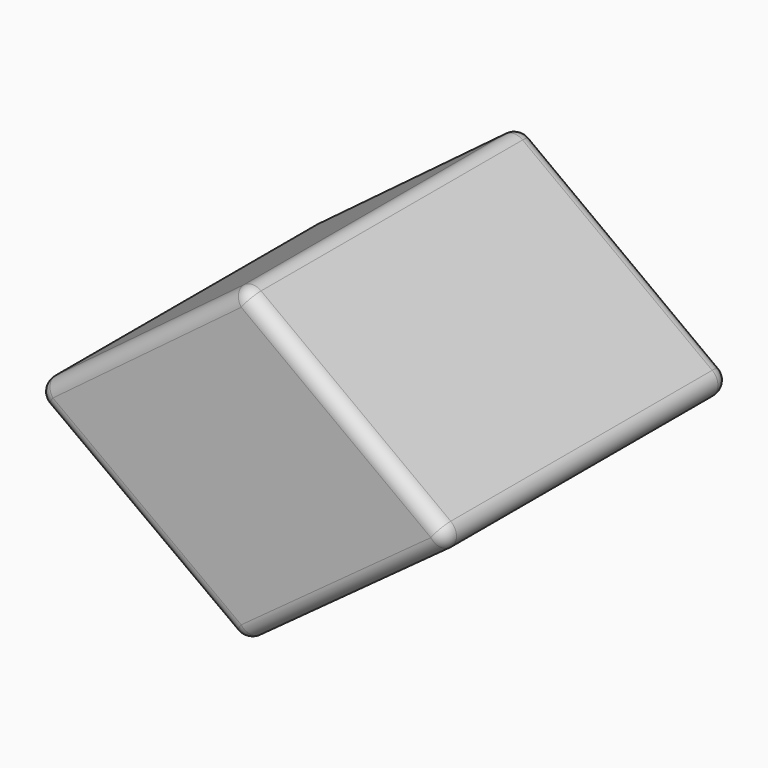
from build123d import *

# Parameters (mm, degrees)
F1_DEPTH       = 25.4
F2_R           = 15.300879685
F3_DEPTH       = 14.478
F4_DEPTH       = 101.6
F6_D           = 13.97
F6_DEPTH       = 76.2
F6_CBORE_D     = 13.97
F6_CBORE_DEPTH = 6.35
F6_TIP         = 4.1970114239
F8_D           = 13.97
F8_DEPTH       = 76.2
F8_CBORE_D     = 13.97
F8_CBORE_DEPTH = 6.35
F8_TIP         = 4.1970114239
F9_R           = 5.08


with BuildPart() as f1:
    # F0 (on Front) → F1 (new body)
    with BuildSketch(Plane.XZ):
        with BuildLine():
            ThreePointArc((-7.1662437988, 0), (-5.0672995858, 5.0672995858), (0, 7.1662437988))
            Line((0, 7.1662437988), (0, 56.8071007729))
            Line((0, 56.8071007729), (-75.8317038417, 0))
            Line((-75.8317038417, 0), (-7.1662437988, 0))
        make_face()
        with BuildLine():
            Line((0, 56.8071007729), (0, 7.1662437988))
            ThreePointArc((0, 7.1662437988), (5.0672995858, 5.0672995858), (7.1662437988, 0))
            Line((7.1662437988, 0), (76.3651058078, 0))
            Line((76.3651058078, 0), (0, 56.8071007729))
        make_face()
        with BuildLine():
            Line((76.3651058078, 0), (7.1662437988, 0))
            ThreePointArc((7.1662437988, 0), (5.0672995858, -5.0672995858), (0, -7.1662437988))
            Line((0, -7.1662437988), (0, -55.740300566))
            Line((0, -55.740300566), (76.3651058078, 0))
        make_face()
        with BuildLine():
            Line((0, -55.740300566), (0, -7.1662437988))
            ThreePointArc((0, -7.1662437988), (-5.0672995858, -5.0672995858), (-7.1662437988, 0))
            Line((-7.1662437988, 0), (-75.8317038417, 0))
            Line((-75.8317038417, 0), (0, -55.740300566))
        make_face()
        with BuildLine():
            Line((7.1662437988, 0), (0, 0))
            Line((0, 0), (0, -7.1662437988))
            ThreePointArc((0, -7.1662437988), (5.0672995858, -5.0672995858), (7.1662437988, 0))
        make_face()
        with BuildLine():
            Line((-7.1662437988, 0), (0, 0))
            Line((0, 0), (0, 7.1662437988))
            ThreePointArc((0, 7.1662437988), (-5.0672995858, 5.0672995858), (-7.1662437988, 0))
        make_face()
        with BuildLine():
            Line((0, 7.1662437988), (0, 0))
            Line((0, 0), (7.1662437988, 0))
            ThreePointArc((7.1662437988, 0), (5.0672995858, 5.0672995858), (0, 7.1662437988))
        make_face()
        with BuildLine():
            Line((0, -7.1662437988), (0, 0))
            Line((0, 0), (-7.1662437988, 0))
            ThreePointArc((-7.1662437988, 0), (-5.0672995858, -5.0672995858), (0, -7.1662437988))
        make_face()
    extrude(amount=F1_DEPTH)

    # F2 (on Front) → F3 (cut)
    with BuildSketch(Plane.XZ):
        Circle(F2_R)
    extrude(amount=F3_DEPTH, mode=Mode.SUBTRACT)

    # F4 (add): a face of the model
    f4_faces = [f1.faces().sort_by_distance(p)[0] for p in [
        (-36.7809633217, 0, 26.8885894929),
    ]]
    extrude(f4_faces, amount=F4_DEPTH)

    # F6
    with Locations(Plane(origin=(0, 101.6, 0), x_dir=(-1, 0, 0), z_dir=(0, 1, 0))):
        with Locations((-45.5900207162, 0)):
            CounterBoreHole(F6_D / 2, F6_CBORE_D / 2, F6_CBORE_DEPTH, depth=F6_DEPTH)
            with Locations((0, 0, -(F6_DEPTH + F6_TIP / 2))):  # 118° drill point
                Cone(0, F6_D / 2, F6_TIP, mode=Mode.SUBTRACT)

    # F8
    with Locations(Plane(origin=(0, 101.6, 0), x_dir=(-1, 0, 0), z_dir=(0, 1, 0))):
        with Locations((45.3492924571, 0)):
            CounterBoreHole(F8_D / 2, F8_CBORE_D / 2, F8_CBORE_DEPTH, depth=F8_DEPTH)
            with Locations((0, 0, -(F8_DEPTH + F8_TIP / 2))):  # 118° drill point
                Cone(0, F8_D / 2, F8_TIP, mode=Mode.SUBTRACT)

    # F9
    f9_edges = [f1.edges().sort_by_distance(p)[0] for p in [
        (38.182553, 101.6, 28.40355),
        (38.182553, 101.6, -27.87015),
        (-15.30088, -14.478, 0),
        (-15.30088, 101.6, 0),
        (-37.915852, -25.4, -27.87015),
        (0, 38.1, -55.740301),
        (-37.915852, 101.6, -27.87015),
        (-75.831704, 38.1, 0),
        (0, 38.1, 56.807101),
        (-37.915852, -25.4, 28.40355),
        (-37.915852, 101.6, 28.40355),
        (38.182553, -25.4, -27.87015),
        (38.182553, -25.4, 28.40355),
        (76.365106, 38.1, 0),
        (-38.364292, 101.6, 0),
        (52.575021, 101.6, 0),
        (-38.364292, 25.4, 0),
        (52.575021, 25.4, 0),
    ]]
    fillet(f9_edges, radius=F9_R)


solid = f1.part
